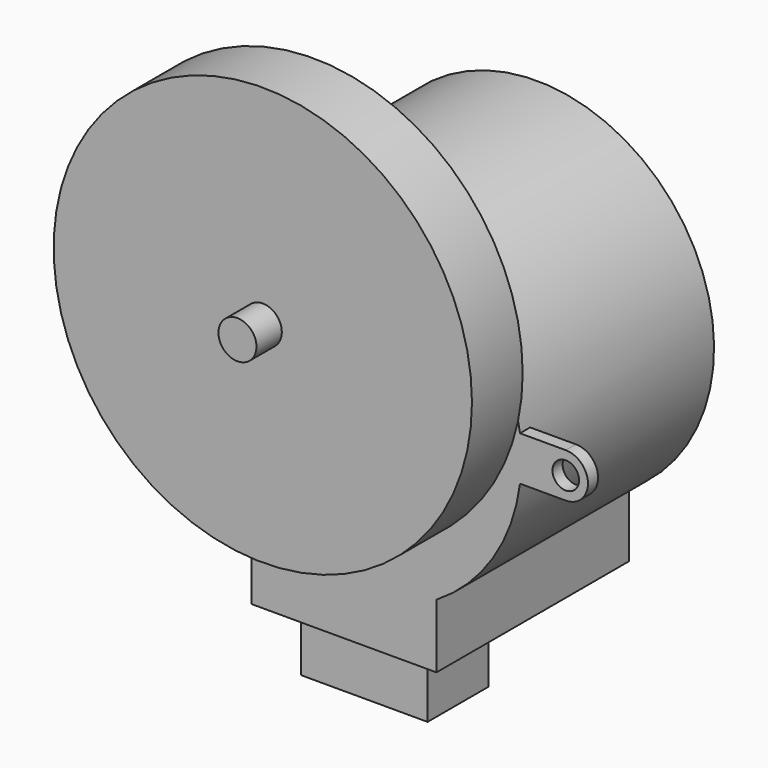
from build123d import *

# Parameters (mm, degrees)
F1_DEPTH  = 19
F2_R      = 3
F3_DEPTH  = 3
F4_R      = 1.5
F5_DEPTH  = 7.5
F6_R      = 1.05
F7_DEPTH  = 1
F8_R      = 16.5
F9_DEPTH  = 5
F10_W     = 10
F10_H     = 6
F11_DEPTH = 5


# Not quite as in the source:
# - a pattern or mirror of a feature is missing from the dataset's text; its kind, count and spacing are read off the source's solid


with BuildPart() as f1:
    # F0 (on Front) → F1 (new body)
    with BuildSketch(Plane.XZ):
        with BuildLine():
            Line((7.3, -17), (7.3, -11.9461290802))
            ThreePointArc((7.3, -11.9461290802), (0, 14), (-7.3, -11.9461290802))
            Line((-7.3, -11.9461290802), (-7.3, -17))
            Line((-7.3, -17), (7.3, -17))
        make_face()
    extrude(amount=F1_DEPTH)

    # F2 (on face) → F3 (join)
    with BuildSketch(Plane.XZ.offset(19)):
        with Locations((0, 8)):
            Circle(F2_R)
    extrude(amount=F3_DEPTH)

    # F4 (on face) → F5 (join)
    with BuildSketch(Plane.XZ.offset(22)):
        with Locations((0, 8)):
            Circle(F4_R)
    extrude(amount=F5_DEPTH)

    # F6 (on face) → F7 (join)
    with BuildSketch(Plane.XZ.offset(19)):
        with BuildLine():
            Line((13.8901943831, -1.75), (17.5, -1.75))
            ThreePointArc((17.5, -1.75), (19.25, 0), (17.5, 1.75))
            Line((17.5, 1.75), (13.8901943831, 1.75))
            Line((13.8901943831, 1.75), (13.8901943831, -1.75))
        make_face()
        with Locations((17.5, 0)):
            Circle(F6_R, mode=Mode.SUBTRACT)
    f7 = extrude(amount=-F7_DEPTH)

    # F7_copies: F7 across plane
    add(f7.mirror(Plane(origin=(0, 0, 0), x_dir=(0, 0, -1), z_dir=(-1, 0, 0))))

    # F8 (on face) → F9 (join)
    with BuildSketch(Plane.XZ.offset(22)):
        with Locations((0, 8)):
            Circle(F8_R)
    extrude(amount=F9_DEPTH)

    # F10 (on face) → F11 (join)
    with BuildSketch(Plane(origin=(0, 0, -17), x_dir=(1, 0, 0), z_dir=(0, 0, -1))):
        with Locations((0, 14)):
            Rectangle(F10_W, F10_H)
    extrude(amount=F11_DEPTH)


solid = f1.part
